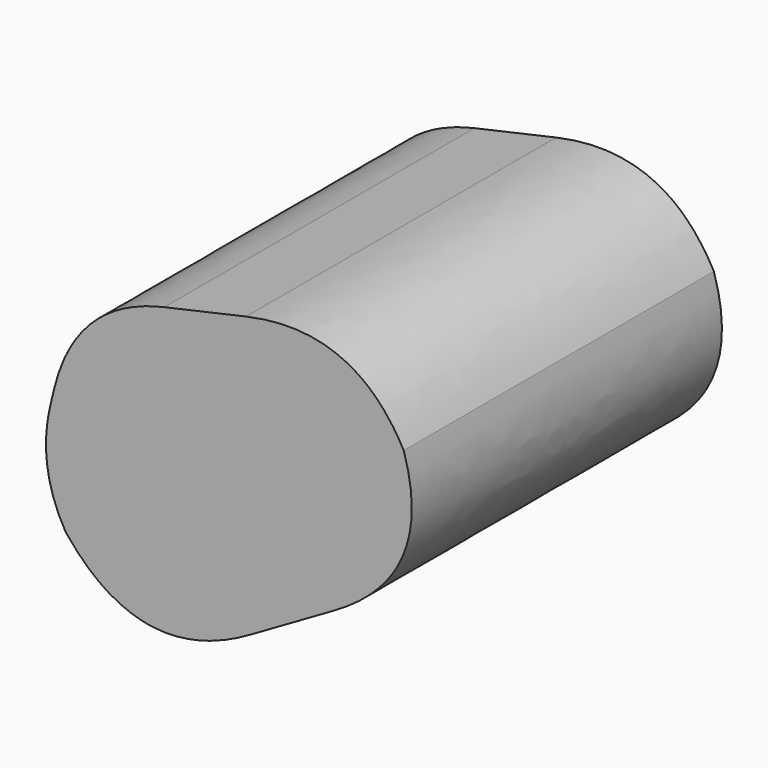
from build123d import *

# Parameters (mm, degrees)
F1_DEPTH    = 67.2322362661
F2_T1_DEPTH = 173.3037820945
F2_T3_DEPTH = 146.4467100197
F2_T5_DEPTH = 179.2908953132
F2_T7_DEPTH = 184.152409541
F2_T9_DEPTH = 124.0966869943


# Not quite as in the source:
# - a fillet or chamfer that OpenCascade refuses, or shapes differently, is made with other operations: its cross-section is extruded or revolved along the edge and cut away or added


with BuildPart() as f1:
    # F0 (on Front) → F1 (new body)
    with BuildSketch(Plane.XZ):
        Polygon((-13.7368068099, -24.4724042714), (40.5815988779, 6.9719441235), (26.5129879117, 40.2553863823), (-23.8238461316, 28.9565175772), (-30.7448208332, 0), align=None)
    extrude(amount=F1_DEPTH)

    # F2: fillet of radius 25.4 on 5 edges, made by hand

    # F2_s2 → F2_t1 (cut)
    with BuildSketch(Plane.XZ.offset(-53.0357729142)):
        with BuildLine():
            add(Edge.make_bspline(
                [(34.7725342315, 20.7149972366), (26.5129879117, 40.2553863823), (5.8137329922, 35.6091234589)],
                knots=[0, 0, 0, 1, 1, 1], degree=2, weights=[1, 1, 1]))
            Line((5.8137329922, 35.6091234589), (26.5129879117, 40.2553863823))
            Line((26.5129879117, 40.2553863823), (34.7725342315, 20.7149972366))
        make_face()
    extrude(amount=F2_T1_DEPTH, mode=Mode.SUBTRACT)

    # F2_s4 → F2_t3 (cut)
    with BuildSketch(Plane.XZ.offset(-39.6072368768)):
        with BuildLine():
            add(Edge.make_bspline(
                [(-8.3655950734, 32.426357387), (-23.8238461316, 28.9565175772), (-27.5067626395, 13.5476422101)],
                knots=[0, 0, 0, 1, 1, 1], degree=2, weights=[1, 1, 1]))
            Line((-27.5067626395, 13.5476422101), (-23.8238461316, 28.9565175772))
            Line((-23.8238461316, 28.9565175772), (-8.3655950734, 32.426357387))
        make_face()
    extrude(amount=F2_T3_DEPTH, mode=Mode.SUBTRACT)

    # F2_s6 → F2_t5 (cut)
    with BuildSketch(Plane.XZ.offset(-56.0293295235)):
        with BuildLine():
            add(Edge.make_bspline(
                [(21.185409412, -4.2563040435), (40.5815988779, 6.9719441235), (31.8558498779, 27.6152729996)],
                knots=[0, 0, 0, 1, 1, 1], degree=2, weights=[1, 1, 1]))
            Line((31.8558498779, 27.6152729996), (40.5815988779, 6.9719441235))
            Line((40.5815988779, 6.9719441235), (21.185409412, -4.2563040435))
        make_face()
    extrude(amount=F2_T5_DEPTH, mode=Mode.SUBTRACT)

    # F2_s8 → F2_t7 (cut)
    with BuildSketch(Plane.XZ.offset(-58.4600866374)):
        with BuildLine():
            add(Edge.make_bspline(
                [(6.5008602522, -12.7570336572), (-13.7368068099, -24.4724042714), (-27.081995831, -5.2703469145)],
                knots=[0, 0, 0, 1, 1, 1], degree=2, weights=[1, 1, 1]))
            Line((-27.081995831, -5.2703469145), (-13.7368068099, -24.4724042714))
            Line((-13.7368068099, -24.4724042714), (6.5008602522, -12.7570336572))
        make_face()
    extrude(amount=F2_T7_DEPTH, mode=Mode.SUBTRACT)

    # F2_s10 → F2_t9 (cut)
    with BuildSketch(Plane.XZ.offset(-28.4322253641)):
        with BuildLine():
            add(Edge.make_bspline(
                [(-28.1010233758, 11.0613274641), (-30.7448208332, 0), (-24.2543511196, -9.3389738816)],
                knots=[0, 0, 0, 1, 1, 1], degree=2, weights=[1, 1, 1]))
            Line((-24.2543511196, -9.3389738816), (-30.7448208332, 0))
            Line((-30.7448208332, 0), (-28.1010233758, 11.0613274641))
        make_face()
    extrude(amount=F2_T9_DEPTH, mode=Mode.SUBTRACT)


solid = f1.part
